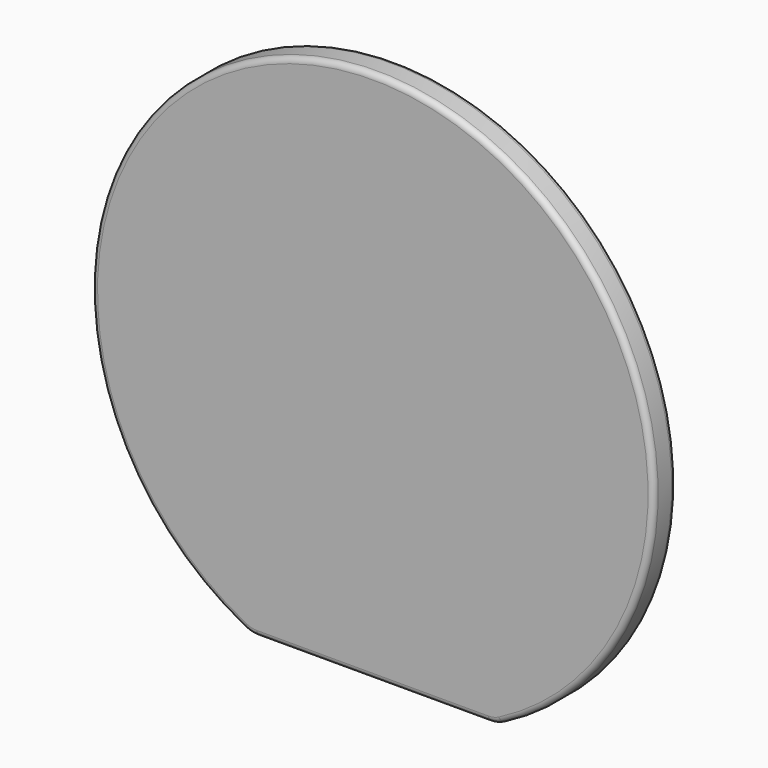
from build123d import *

# Parameters (mm, degrees)
F1_DEPTH = 5
F2_R     = 5
F3_R     = 1


with BuildPart() as f1:
    # F0 (on Front) → F1 (new body)
    with BuildSketch(Plane.XZ):
        with BuildLine():
            Line((-21.7944947177, -45), (21.7944947177, -45))
            ThreePointArc((21.7944947177, -45), (0, 50), (-21.7944947177, -45))
        make_face()
    extrude(amount=F1_DEPTH)

    # F2
    f2_edges = [f1.edges().sort_by_distance(p)[0] for p in [
        (21.794495, -2.5, -45),
        (-21.794495, -2.5, -45),
    ]]
    fillet(f2_edges, radius=F2_R)

    # F3
    f3_edges = [f1.edges().sort_by_distance(p)[0] for p in [
        (0, -5, 50),
        (0, 0, 50),
        (0, -5, -45),
        (0, 0, -45),
        (-21.794039, 0, -44.859127),
        (21.794039, 0, -44.859127),
        (-21.794039, -5, -44.859127),
        (21.794039, -5, -44.859127),
    ]]
    fillet(f3_edges, radius=F3_R)


solid = f1.part
